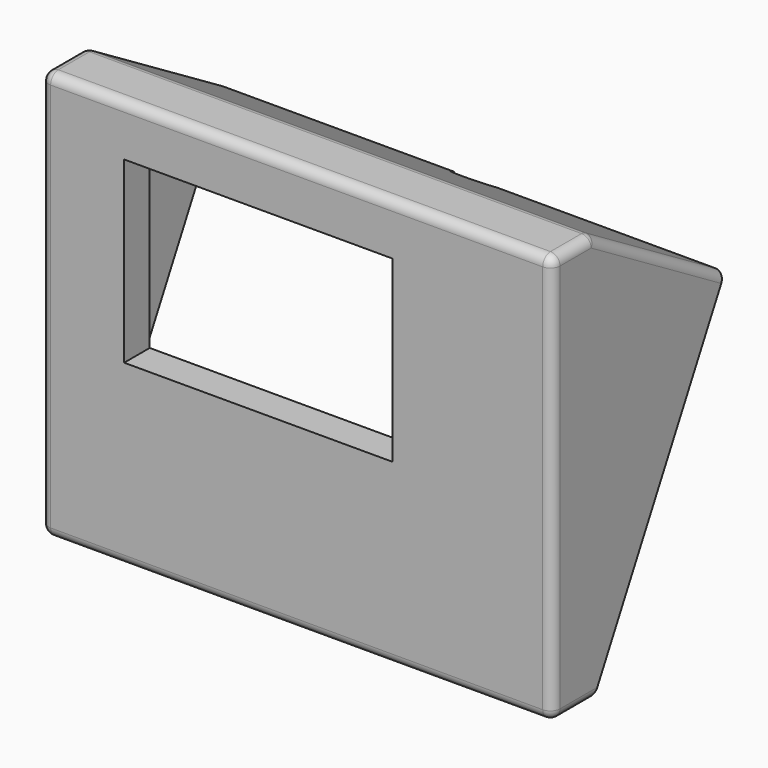
from build123d import *

# Parameters (mm, degrees)
F0_W      = 80
F0_H      = 64
F0_W_2    = 42
F0_H_2    = 28
F1_DEPTH  = 3
F4_DEPTH  = 80
F5_T      = -2
F6_DEPTH  = 5
F7_R      = 1.5
F12_DEPTH = 2
F13_DEPTH = 2
F15_R     = 3.3298156999
F16_DEPTH = 25


# Not quite as in the source:
# - a feature names something its author has since deleted; it is built from what else it names


with BuildPart() as f1:
    # F0 (on Front) → F1 (new body)
    with BuildSketch(Plane.XZ):
        with Locations((-1, 1.9610269163)):
            Rectangle(F0_W, F0_H)
        with Locations((-7, 11.9610269163)):
            Rectangle(F0_W_2, F0_H_2, mode=Mode.SUBTRACT)
    extrude(amount=F1_DEPTH)

    # F3 (on offset) → F4 (join)
    with BuildSketch(Plane(origin=(-41, 0, 0), x_dir=(0, -1, 0), z_dir=(-1, 0, 0))):
        Polygon((0, -30.0389730837), (0, 33.9610269163), (-5, 33.9610269163), (-30.7466138076, 18.5625894163), (-5, -30.0389730837), align=None)
    extrude(amount=-F4_DEPTH)

    # F5
    f5_openings = [f1.faces().sort_by_distance(p)[0] for p in [
        (-1, 17.873307, -5.738192),
    ]]
    offset(amount=F5_T, openings=f5_openings, kind=Kind.INTERSECTION)

    # F0 (on Front) → F6 (cut)
    with BuildSketch(Plane.XZ):
        with Locations((-7, 11.9610269163)):
            Rectangle(F0_W_2, F0_H_2)
    extrude(amount=-F6_DEPTH, mode=Mode.SUBTRACT)

    # F7
    f7_edges = [f1.edges().sort_by_distance(p)[0] for p in [
        (39, -3, 1.961027),
        (39, 1, -30.038973),
        (-1, -3, -30.038973),
        (39, 1, 33.961027),
        (39, 17.873307, 26.261808),
        (-1, -3, 33.961027),
        (-1, 5, 33.961027),
        (-41, -3, 1.961027),
        (-41, 1, 33.961027),
        (-41, 17.873307, 26.261808),
        (-41, 1, -30.038973),
    ]]
    fillet(f7_edges, radius=F7_R)


with BuildPart() as f8_1:
    # F8: copy of F1
    add(f1.part)


with BuildPart() as f1_1:
    add(f1.part)

    # F11 (on offset) → F12 (join)
    with BuildSketch(Plane(origin=(0, 16.3302800697, -8.6509443873), x_dir=(-1, 0, 0), z_dir=(0, 0.8836647727, -0.468120251))):
        Polygon((-37, -15.9132964909), (-37, -21.9031590968), (39, -21.8151584268), (39, -15.9132964909), align=None)
    extrude(amount=-F12_DEPTH)

    # F11 (on offset) → F13 (join)
    with BuildSketch(Plane(origin=(0, 16.3302800697, -8.6509443873), x_dir=(-1, 0, 0), z_dir=(0, 0.8836647727, -0.468120251))):
        Polygon((39, 22.7937423885), (39, 28.7937423885), (-37, 28.7524405867), (-37, 22.7937423885), align=None)
    extrude(amount=-F13_DEPTH)

    # F15 (on offset) → F16 (cut)
    with BuildSketch(Plane(origin=(0, 16.2774082354, 27.2162772116), x_dir=(1, 0, 0), z_dir=(0, 0.51328125, 0.8582204603))):
        with Locations((0, 16.920266673)):
            Circle(F15_R)
    extrude(amount=-F16_DEPTH, mode=Mode.SUBTRACT)


solid = f1_1.part
